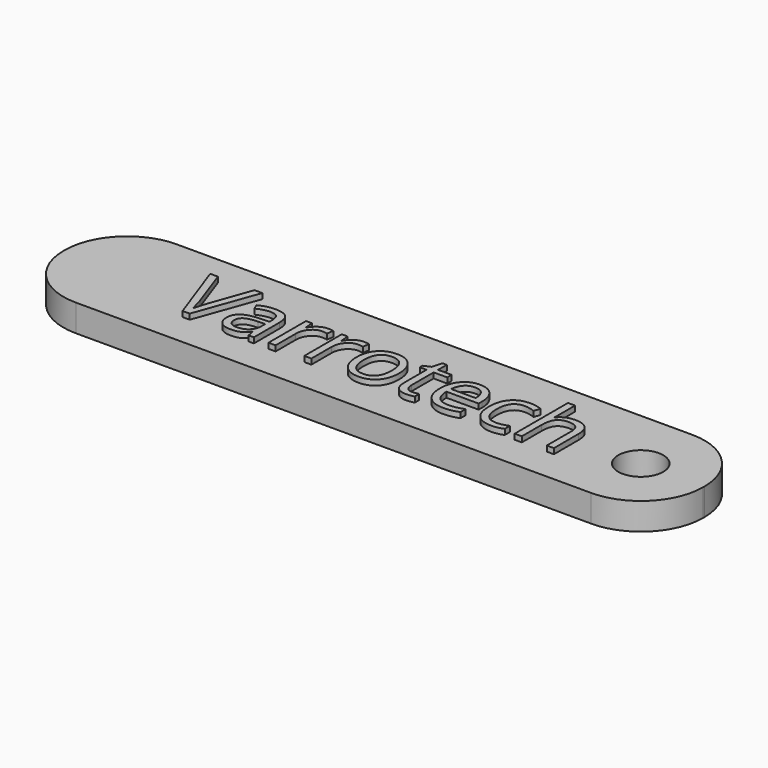
from build123d import *

# Parameters (mm, degrees)
F0_W         = 71
F0_H         = 14
F0_R         = 2.5
F1_DEPTH     = 3
F2_R         = 6.9
F3_TEXT_SIZE = 9.7222222222
F4_DEPTH     = 0.6


# Not quite as in the source:
# - Text() gives the source's letters only with a copy of the font that has no kerning and outlines rounded to 1/6400 em; it was checked with that copy


with BuildPart() as f1:
    # F0 (on Top) → F1 (new body)
    with BuildSketch(Plane.XY):
        Rectangle(F0_W, F0_H)
        with Locations((28.5, 0)):
            Circle(F0_R, mode=Mode.SUBTRACT)
    extrude(amount=F1_DEPTH)

    # F2
    f2_edges = [f1.edges().sort_by_distance(p)[0] for p in [
        (35.5, -7, 1.5),
        (35.5, 7, 1.5),
        (-35.5, -7, 1.5),
        (-35.5, 7, 1.5),
    ]]
    fillet(f2_edges, radius=F2_R)

    # F3 (on face) → F4 (join)
    with BuildSketch(Plane.XY.offset(3)):
        with Locations((-22.1674262153, -3.3494612251)):
            Text('Varrotech', F3_TEXT_SIZE, font='Open Sans', text_align=(TextAlign.LEFT, TextAlign.BOTTOM))
    extrude(amount=F4_DEPTH)


solid = f1.part
